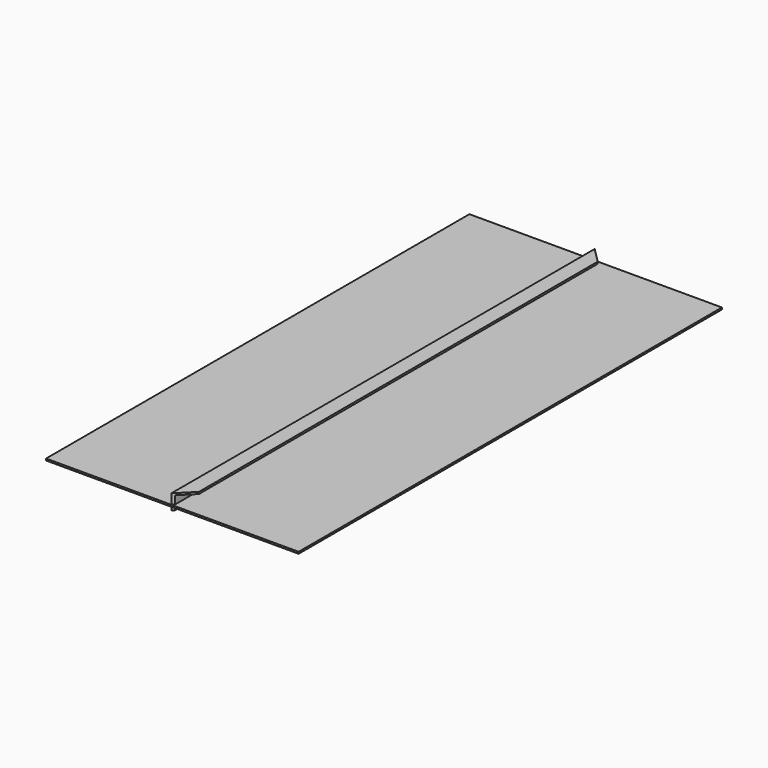
from build123d import *

# Parameters (mm, degrees)
F1_DEPTH = 440
F3_DEPTH = 25.4
F4_W     = 420
F4_H     = 880
F5_DEPTH = 1.5


# Not quite as in the source:
# - a pattern or mirror of a feature is missing from the dataset's text; its kind, count and spacing are read off the source's solid


with BuildPart() as f1:
    # F0 (on Front) → F1 (new body, symmetric)
    with BuildSketch(Plane.XZ):
        Polygon((1.6, -7.0391468048), (1.6, 15.1606531952), (23.7998, 15.1606531952), (23.7998, 18.3608531952), (-1.6002, 18.3608531952), (-1.6002, -7.0391468048), align=None)
    extrude(amount=F1_DEPTH, both=True)

    # F2 (on face) → F3 (cut)
    with BuildSketch(Plane.XY.offset(18.3608531952)):
        Polygon((23.7998, -414.6), (-1.6002, -440), (23.7998, -440), align=None)
    f3 = extrude(amount=-F3_DEPTH, mode=Mode.SUBTRACT)

    # F3_copies: F3 across plane
    add(f3.mirror(Plane.ZX), mode=Mode.SUBTRACT)


with BuildPart() as f5:
    # F4 (on Top) → F5 (new body, symmetric)
    with BuildSketch(Plane.XY):
        Rectangle(F4_W, F4_H)
    extrude(amount=F5_DEPTH, both=True)


solid = Compound([f1.part, f5.part])
